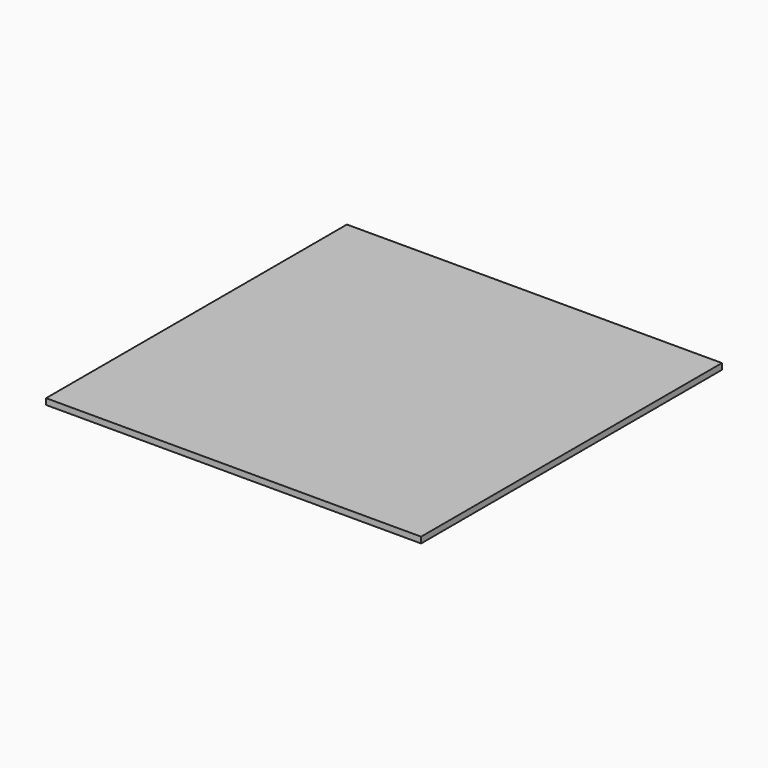
from build123d import *

# Parameters (mm, degrees)
F0_W     = 199.451291883
F0_H     = 200
F1_DEPTH = 3.2


# Not quite as in the source:
# - the program builds the solid bodies; features that only make, move or delete a surface that nothing else refers to are left out


with BuildPart() as f1:
    # F0 (on Top) → F1 (new body)
    with BuildSketch(Plane.XY):
        with Locations((-0.1037493348, -0.3111958504)):
            Rectangle(F0_W, F0_H)
    extrude(amount=F1_DEPTH)


solid = f1.part
